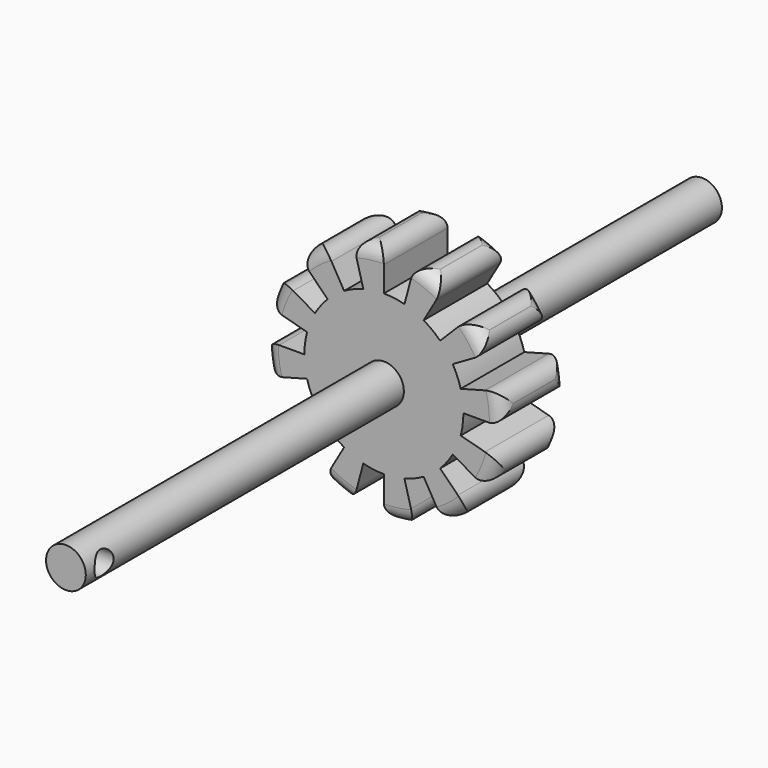
from build123d import *

# Parameters (mm, degrees)
F1_DEPTH      = 12.7
F2_R          = 2.1844
F3_R          = 3.175
F4_DEPTH      = 63.5
F4_DEPTH_BACK = 63.5
F5_R          = 1.905
F6_DEPTH      = 6.35
F6_DEPTH_BACK = 6.35


with BuildPart() as f1:
    # F0 (on Front) → F1 (new body)
    with BuildSketch(Plane.XZ):
        with BuildLine():
            Line((6.3329836945, -10.9762801945), (-0.0170163055, 0.0222424335))
            Line((-0.0170163055, 0.0222424335), (3.2699855673, -12.2450155604))
            ThreePointArc((3.2699855673, -12.2450155604), (4.8430632856, -11.7110276294), (6.3329836945, -10.9762801945))
        make_face()
        with BuildLine():
            Line((-0.0170163055, -12.6777575665), (-0.0170163055, 0.0222424335))
            Line((-0.0170163055, 0.0222424335), (-3.3040181783, -12.2450155604))
            ThreePointArc((-3.3040181783, -12.2450155604), (-1.6746989467, -12.5691073059), (-0.0170163055, -12.6777575665))
        make_face()
        with BuildLine():
            Line((-6.3670163055, -10.9762801945), (-0.0170163055, 0.0222424335))
            Line((-0.0170163055, 0.0222424335), (-8.9972724265, -8.9580136876))
            ThreePointArc((-8.9972724265, -8.9580136876), (-7.7482864539, -10.0533449882), (-6.3670163055, -10.9762801945))
        make_face()
        with BuildLine():
            Line((-11.0155389335, -6.3277575665), (-0.0170163055, 0.0222424335))
            Line((-0.0170163055, 0.0222424335), (-12.2842742993, -3.2647594393))
            ThreePointArc((-12.2842742993, -3.2647594393), (-11.7502863684, -4.8378371575), (-11.0155389335, -6.3277575665))
        make_face()
        with BuildLine():
            Line((-8.9972724265, -8.9580136876), (-0.0170163055, 0.0222424335))
            Line((-0.0170163055, 0.0222424335), (-11.0155389335, -6.3277575665))
            ThreePointArc((-11.0155389335, -6.3277575665), (-10.0926037272, -7.7090277149), (-8.9972724265, -8.9580136876))
        make_face()
        with BuildLine():
            Line((-3.3040181783, -12.2450155604), (-0.0170163055, 0.0222424335))
            Line((-0.0170163055, 0.0222424335), (-6.3670163055, -10.9762801945))
            ThreePointArc((-6.3670163055, -10.9762801945), (-4.8770958965, -11.7110276294), (-3.3040181783, -12.2450155604))
        make_face()
        with BuildLine():
            Line((3.2699855673, -12.2450155604), (-0.0170163055, 0.0222424335))
            Line((-0.0170163055, 0.0222424335), (-0.0170163055, -12.6777575665))
            ThreePointArc((-0.0170163055, -12.6777575665), (1.6406663357, -12.5691073059), (3.2699855673, -12.2450155604))
        make_face()
        with BuildLine():
            Line((8.9632398156, -8.9580136876), (-0.0170163055, 0.0222424335))
            Line((-0.0170163055, 0.0222424335), (6.3329836945, -10.9762801945))
            ThreePointArc((6.3329836945, -10.9762801945), (7.7142538429, -10.0533449882), (8.9632398156, -8.9580136876))
        make_face()
        with BuildLine():
            Line((10.9815063226, -6.3277575665), (-0.0170163055, 0.0222424335))
            Line((-0.0170163055, 0.0222424335), (8.9632398156, -8.9580136876))
            ThreePointArc((8.9632398156, -8.9580136876), (10.0585711162, -7.7090277149), (10.9815063226, -6.3277575665))
        make_face()
        with BuildLine():
            ThreePointArc((10.9815063226, -6.3277575665), (11.7162537574, -4.8378371575), (12.2502416884, -3.2647594393))
            Line((12.2502416884, -3.2647594393), (-0.0170163055, 0.0222424335))
            Line((-0.0170163055, 0.0222424335), (10.9815063226, -6.3277575665))
        make_face()
        with BuildLine():
            ThreePointArc((12.2502416884, -3.2647594393), (12.574333434, -1.6354402077), (12.6829836945, 0.0222424335))
            Line((12.6829836945, 0.0222424335), (-0.0170163055, 0.0222424335))
            Line((-0.0170163055, 0.0222424335), (12.2502416884, -3.2647594393))
        make_face()
        with BuildLine():
            Line((-0.0170163055, 0.0222424335), (12.6829836945, 0.0222424335))
            ThreePointArc((12.6829836945, 0.0222424335), (12.574333434, 1.6799250747), (12.2502416884, 3.3092443063))
            Line((12.2502416884, 3.3092443063), (-0.0170163055, 0.0222424335))
        make_face()
        with BuildLine():
            Line((-0.0170163055, 0.0222424335), (12.2502416884, 3.3092443063))
            ThreePointArc((12.2502416884, 3.3092443063), (11.7162537574, 4.8823220246), (10.9815063226, 6.3722424335))
            Line((10.9815063226, 6.3722424335), (-0.0170163055, 0.0222424335))
        make_face()
        with BuildLine():
            Line((8.9632398156, 9.0024985546), (-0.0170163055, 0.0222424335))
            Line((-0.0170163055, 0.0222424335), (10.9815063226, 6.3722424335))
            ThreePointArc((10.9815063226, 6.3722424335), (10.0585711162, 7.7535125819), (8.9632398156, 9.0024985546))
        make_face()
        with BuildLine():
            Line((6.3329836945, 11.0207650616), (-0.0170163055, 0.0222424335))
            Line((-0.0170163055, 0.0222424335), (8.9632398156, 9.0024985546))
            ThreePointArc((8.9632398156, 9.0024985546), (7.7142538429, 10.0978298552), (6.3329836945, 11.0207650616))
        make_face()
        with BuildLine():
            Line((3.2699855673, 12.2895004274), (-0.0170163055, 0.0222424335))
            Line((-0.0170163055, 0.0222424335), (6.3329836945, 11.0207650616))
            ThreePointArc((6.3329836945, 11.0207650616), (4.8430632856, 11.7555124964), (3.2699855673, 12.2895004274))
        make_face()
        with BuildLine():
            Line((-0.0170163055, 12.7222424335), (-0.0170163055, 0.0222424335))
            Line((-0.0170163055, 0.0222424335), (3.2699855673, 12.2895004274))
            ThreePointArc((3.2699855673, 12.2895004274), (1.6406663357, 12.613592173), (-0.0170163055, 12.7222424335))
        make_face()
        with BuildLine():
            Line((-3.3040181783, 12.2895004274), (-0.0170163055, 0.0222424335))
            Line((-0.0170163055, 0.0222424335), (-0.0170163055, 12.7222424335))
            ThreePointArc((-0.0170163055, 12.7222424335), (-1.6746989467, 12.613592173), (-3.3040181783, 12.2895004274))
        make_face()
        with BuildLine():
            Line((-6.3670163055, 11.0207650616), (-0.0170163055, 0.0222424335))
            Line((-0.0170163055, 0.0222424335), (-3.3040181783, 12.2895004274))
            ThreePointArc((-3.3040181783, 12.2895004274), (-4.8770958965, 11.7555124964), (-6.3670163055, 11.0207650616))
        make_face()
        with BuildLine():
            Line((-8.9972724265, 9.0024985546), (-0.0170163055, 0.0222424335))
            Line((-0.0170163055, 0.0222424335), (-6.3670163055, 11.0207650616))
            ThreePointArc((-6.3670163055, 11.0207650616), (-7.7482864539, 10.0978298552), (-8.9972724265, 9.0024985546))
        make_face()
        with BuildLine():
            Line((-11.0155389335, 6.3722424335), (-0.0170163055, 0.0222424335))
            Line((-0.0170163055, 0.0222424335), (-8.9972724265, 9.0024985546))
            ThreePointArc((-8.9972724265, 9.0024985546), (-10.0926037272, 7.7535125819), (-11.0155389335, 6.3722424335))
        make_face()
        with BuildLine():
            Line((-12.2842742993, 3.3092443063), (-0.0170163055, 0.0222424335))
            Line((-0.0170163055, 0.0222424335), (-11.0155389335, 6.3722424335))
            ThreePointArc((-11.0155389335, 6.3722424335), (-11.7502863684, 4.8823220246), (-12.2842742993, 3.3092443063))
        make_face()
        with BuildLine():
            Line((-12.7170163055, 0.0222424335), (-0.0170163055, 0.0222424335))
            Line((-0.0170163055, 0.0222424335), (-12.2842742993, 3.3092443063))
            ThreePointArc((-12.2842742993, 3.3092443063), (-12.6083660449, 1.6799250747), (-12.7170163055, 0.0222424335))
        make_face()
        with BuildLine():
            Line((-12.2842742993, -3.2647594393), (-0.0170163055, 0.0222424335))
            Line((-0.0170163055, 0.0222424335), (-12.7170163055, 0.0222424335))
            ThreePointArc((-12.7170163055, 0.0222424335), (-12.6083660449, -1.6354402077), (-12.2842742993, -3.2647594393))
        make_face()
        with BuildLine():
            ThreePointArc((-12.2842742993, 3.3092443063), (-11.7502863684, 4.8823220246), (-11.0155389335, 6.3722424335))
            Line((-11.0155389335, 6.3722424335), (-16.5148002476, 9.5472424335))
            ThreePointArc((-16.5148002476, 9.5472424335), (-17.6169213998, 7.3123618201), (-18.4179032963, 4.9527452427))
            Line((-18.4179032963, 4.9527452427), (-12.2842742993, 3.3092443063))
        make_face()
        with BuildLine():
            Line((-18.4179032963, -4.9082603757), (-12.2842742993, -3.2647594393))
            ThreePointArc((-12.2842742993, -3.2647594393), (-12.6083660449, -1.6354402077), (-12.7170163055, 0.0222424335))
            Line((-12.7170163055, 0.0222424335), (-19.0670163055, 0.0222424335))
            ThreePointArc((-19.0670163055, 0.0222424335), (-18.9040409146, -2.4642815283), (-18.4179032963, -4.9082603757))
        make_face()
        with BuildLine():
            Line((-13.4874004871, -13.4481417481), (-8.9972724265, -8.9580136876))
            ThreePointArc((-8.9972724265, -8.9580136876), (-10.0926037272, -7.7090277149), (-11.0155389335, -6.3277575665))
            Line((-11.0155389335, -6.3277575665), (-16.5148002476, -9.5027575665))
            ThreePointArc((-16.5148002476, -9.5027575665), (-15.130397438, -11.5746627891), (-13.4874004871, -13.4481417481))
        make_face()
        with BuildLine():
            Line((-4.9475191147, -18.3786445573), (-3.3040181783, -12.2450155604))
            ThreePointArc((-3.3040181783, -12.2450155604), (-4.8770958965, -11.7110276294), (-6.3670163055, -10.9762801945))
            Line((-6.3670163055, -10.9762801945), (-9.5420163055, -16.4755415086))
            ThreePointArc((-9.5420163055, -16.4755415086), (-7.307135692, -17.5776626608), (-4.9475191147, -18.3786445573))
        make_face()
        with BuildLine():
            Line((18.3838706853, -4.9082603757), (12.2502416884, -3.2647594393))
            ThreePointArc((12.2502416884, -3.2647594393), (11.7162537574, -4.8378371575), (10.9815063226, -6.3277575665))
            Line((10.9815063226, -6.3277575665), (16.4807676366, -9.5027575665))
            ThreePointArc((16.4807676366, -9.5027575665), (17.5828887889, -7.267876953), (18.3838706853, -4.9082603757))
        make_face()
        with BuildLine():
            ThreePointArc((12.2502416884, 3.3092443063), (12.574333434, 1.6799250747), (12.6829836945, 0.0222424335))
            Line((12.6829836945, 0.0222424335), (19.0329836945, 0.0222424335))
            ThreePointArc((19.0329836945, 0.0222424335), (18.8700083037, 2.5087663953), (18.3838706853, 4.9527452427))
            Line((18.3838706853, 4.9527452427), (12.2502416884, 3.3092443063))
        make_face()
        with BuildLine():
            ThreePointArc((8.9632398156, 9.0024985546), (10.0585711162, 7.7535125819), (10.9815063226, 6.3722424335))
            Line((10.9815063226, 6.3722424335), (16.4807676366, 9.5472424335))
            ThreePointArc((16.4807676366, 9.5472424335), (15.0963648271, 11.6191476561), (13.4533678761, 13.4926266151))
            Line((13.4533678761, 13.4926266151), (8.9632398156, 9.0024985546))
        make_face()
        with BuildLine():
            Line((4.9134865037, 18.4231294243), (3.2699855673, 12.2895004274))
            ThreePointArc((3.2699855673, 12.2895004274), (4.8430632856, 11.7555124964), (6.3329836945, 11.0207650616))
            Line((6.3329836945, 11.0207650616), (9.5079836945, 16.5200263756))
            ThreePointArc((9.5079836945, 16.5200263756), (7.2731030811, 17.6221475279), (4.9134865037, 18.4231294243))
        make_face()
        with BuildLine():
            ThreePointArc((-3.3040181783, 12.2895004274), (-1.6746989467, 12.613592173), (-0.0170163055, 12.7222424335))
            Line((-0.0170163055, 12.7222424335), (-0.0170163055, 19.0722424335))
            ThreePointArc((-0.0170163055, 19.0722424335), (-2.5035402673, 18.9092670427), (-4.9475191147, 18.4231294243))
            Line((-4.9475191147, 18.4231294243), (-3.3040181783, 12.2895004274))
        make_face()
        with BuildLine():
            Line((-13.4874004871, 13.4926266151), (-8.9972724265, 9.0024985546))
            ThreePointArc((-8.9972724265, 9.0024985546), (-7.7482864539, 10.0978298552), (-6.3670163055, 11.0207650616))
            Line((-6.3670163055, 11.0207650616), (-9.5420163055, 16.5200263756))
            ThreePointArc((-9.5420163055, 16.5200263756), (-11.6139215281, 15.1356235661), (-13.4874004871, 13.4926266151))
        make_face()
        with BuildLine():
            Line((4.9134865037, -18.3786445573), (3.2699855673, -12.2450155604))
            ThreePointArc((3.2699855673, -12.2450155604), (1.6406663357, -12.5691073059), (-0.0170163055, -12.6777575665))
            Line((-0.0170163055, -12.6777575665), (-0.0170163055, -19.0277575665))
            ThreePointArc((-0.0170163055, -19.0277575665), (2.4695076563, -18.8647821757), (4.9134865037, -18.3786445573))
        make_face()
        with BuildLine():
            Line((13.4533678761, -13.4481417481), (8.9632398156, -8.9580136876))
            ThreePointArc((8.9632398156, -8.9580136876), (7.7142538429, -10.0533449882), (6.3329836945, -10.9762801945))
            Line((6.3329836945, -10.9762801945), (9.5079836945, -16.4755415086))
            ThreePointArc((9.5079836945, -16.4755415086), (11.5798889172, -15.091138699), (13.4533678761, -13.4481417481))
        make_face()
    extrude(amount=F1_DEPTH)

    # F2
    f2_edges = [f1.edges().sort_by_distance(p)[0] for p in [
        (9.507984, -6.35, -16.475542),
        (13.453368, -6.35, -13.448142),
        (11.579889, 0, -15.091139),
        (11.579889, -12.7, -15.091139),
        (16.480768, -6.35, -9.502758),
        (18.383871, -6.35, -4.90826),
        (17.582889, 0, -7.267877),
        (17.582889, -12.7, -7.267877),
        (-0.017016, -6.35, -19.027758),
        (4.913487, -6.35, -18.378645),
        (2.469508, 0, -18.864782),
        (2.469508, -12.7, -18.864782),
        (19.032984, -6.35, 0.022242),
        (18.383871, -6.35, 4.952745),
        (18.870008, 0, 2.508766),
        (18.870008, -12.7, 2.508766),
        (16.480768, -6.35, 9.547242),
        (13.453368, -6.35, 13.492627),
        (15.096365, 0, 11.619148),
        (15.096365, -12.7, 11.619148),
        (9.507984, -6.35, 16.520026),
        (4.913487, -6.35, 18.423129),
        (7.273103, 0, 17.622148),
        (7.273103, -12.7, 17.622148),
        (-0.017016, -6.35, 19.072242),
        (-4.947519, -6.35, 18.423129),
        (-2.50354, 0, 18.909267),
        (-2.50354, -12.7, 18.909267),
        (-9.542016, -6.35, 16.520026),
        (-13.4874, -6.35, 13.492627),
        (-11.613922, 0, 15.135624),
        (-11.613922, -12.7, 15.135624),
        (-16.5148, -6.35, 9.547242),
        (-18.417903, -6.35, 4.952745),
        (-17.616921, 0, 7.312362),
        (-17.616921, -12.7, 7.312362),
        (-19.067016, -6.35, 0.022242),
        (-18.417903, -6.35, -4.90826),
        (-18.904041, 0, -2.464282),
        (-18.904041, -12.7, -2.464282),
        (-16.5148, -6.35, -9.502758),
        (-13.4874, -6.35, -13.448142),
        (-15.130397, 0, -11.574663),
        (-15.130397, -12.7, -11.574663),
        (-9.542016, -6.35, -16.475542),
        (-4.947519, -6.35, -18.378645),
        (-7.307136, 0, -17.577663),
        (-7.307136, -12.7, -17.577663),
    ]]
    fillet(f2_edges, radius=F2_R)

    # F3 (on face) → F4 (join, two sides)
    with BuildSketch(Plane.XZ.offset(12.7)) as f4_sk:
        Circle(F3_R)
    extrude(amount=F4_DEPTH)
    extrude(f4_sk.sketch, amount=-F4_DEPTH_BACK)

    # F5 (on Right) → F6 (cut, two sides)
    with BuildSketch(Plane.YZ) as f6_sk:
        with Locations((-72.5358724594, 0)):
            Circle(F5_R)
    extrude(amount=F6_DEPTH, mode=Mode.SUBTRACT)
    extrude(f6_sk.sketch, amount=-F6_DEPTH_BACK, mode=Mode.SUBTRACT)


solid = f1.part
